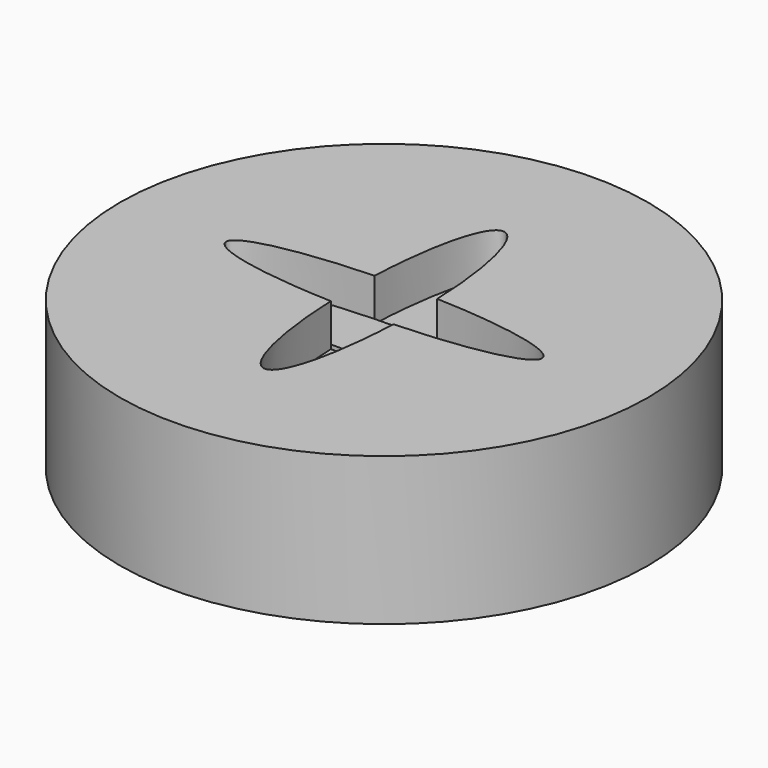
from build123d import *

# Parameters (mm, degrees)
F0_R     = 31.75
F1_DEPTH = 17.78
F2_R     = 25.908
F3_DEPTH = 10.16
F5_DEPTH = 4.572
F7_DEPTH = 5.08


with BuildPart() as f1:
    # F0 (on Top) → F1 (new body)
    with BuildSketch(Plane.XY):
        Circle(F0_R)
    extrude(amount=F1_DEPTH)

    # F2 (on face) → F3 (cut)
    with BuildSketch(Plane(origin=(0, 0, 0), x_dir=(1, 0, 0), z_dir=(0, 0, -1))):
        Circle(F2_R)
    extrude(amount=-F3_DEPTH, mode=Mode.SUBTRACT)

    # F4 (on face) → F5 (cut)
    with BuildSketch(Plane.XY.offset(17.78)):
        with BuildLine():
            add(Edge.make_bspline(
                [(-18.9828891307, 0), (-18.9828891307, -5.8255543832), (9.4914445654, -2.9127771916), (37.9657782614, 0), (9.4914445654, 2.9127771916), (-18.9828891307, 5.8255543832), (-18.9828891307, 0)],
                knots=[0, 0, 0, 2.0943951024, 2.0943951024, 4.1887902048, 4.1887902048, 6.2831853072, 6.2831853072, 6.2831853072], degree=2, weights=[1, 0.5, 1, 0.5, 1, 0.5, 1]))
        make_face()
    extrude(amount=-F5_DEPTH, mode=Mode.SUBTRACT)

    # F6 (on face) → F7 (cut)
    with BuildSketch(Plane.XY.offset(17.78)):
        with BuildLine():
            add(Edge.make_bspline(
                [(3.7629278729, 3.2966425981), (3.177786528, 17.9034117609), (0, 17.9034117609)],
                knots=[4.8975806012, 4.8975806012, 4.8975806012, 6.2831853072, 6.2831853072, 6.2831853072], degree=2, weights=[1, 0.7694591871, 1]))
            add(Edge.make_bspline(
                [(0, 17.9034117609), (-3.177786528, 17.9034117609), (-3.7629278729, 3.2966425981)],
                knots=[0, 0, 0, 1.385604706, 1.385604706, 1.385604706], degree=2, weights=[1, 0.7694591871, 1]))
            add(Edge.make_bspline(
                [(3.7629278729, 3.2966425981), (0, 3.4314794382), (-3.7629278729, 3.2966425981)],
                knots=[4.5500073421, 4.5500073421, 4.5500073421, 4.9395082154, 4.9395082154, 4.9395082154], degree=2, weights=[0.8572768974, 0.7963648883, 0.770038824]))
        make_face()
        with BuildLine():
            add(Edge.make_bspline(
                [(-3.7629278729, -3.2966425981), (0, -3.4314794382), (3.7629278729, -3.2966425981)],
                knots=[1.3436770918, 1.3436770918, 1.3436770918, 1.7331779651, 1.7331779651, 1.7331779651], degree=2, weights=[0.770038824, 0.7963648883, 0.8572768974]))
            add(Edge.make_bspline(
                [(-3.7629278729, -3.2966425981), (-3.177786528, -17.9034117609), (0, -17.9034117609), (3.177786528, -17.9034117609), (3.7629278729, -3.2966425981)],
                knots=[1.7559879476, 1.7559879476, 1.7559879476, 3.1415926536, 3.1415926536, 4.5271973595, 4.5271973595, 4.5271973595], degree=2, weights=[1, 0.7694591871, 1, 0.7694591871, 1]))
        make_face()
    extrude(amount=-F7_DEPTH, mode=Mode.SUBTRACT)


solid = f1.part
